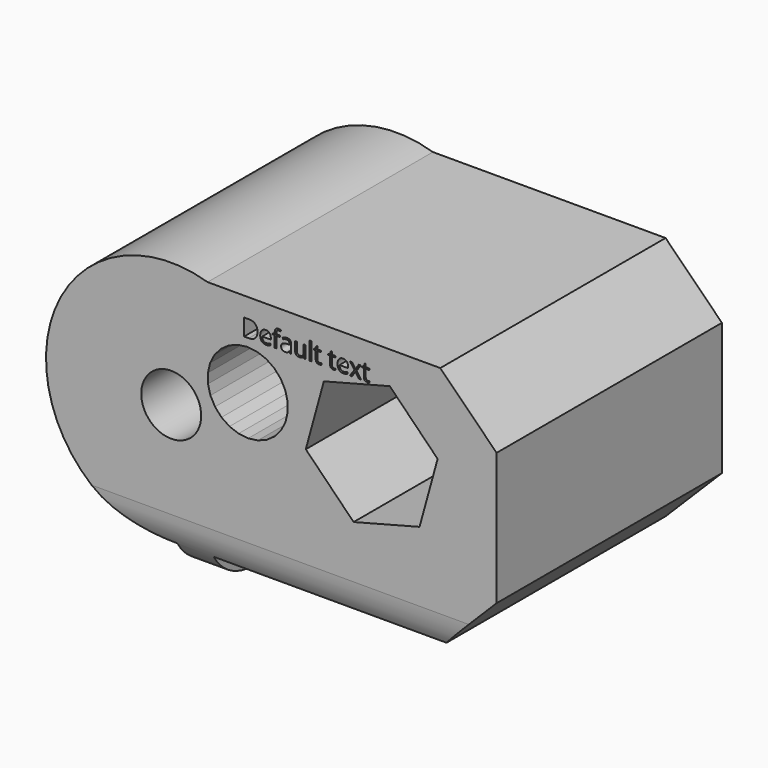
from build123d import *

# Parameters (mm, degrees)
F0_R     = 2.7024697733
F0_W     = 0.1718478913
F0_H     = 1.6102048079
F1_DEPTH = 25.4
F2_SIZE  = 5.08
F3_R     = 5.08


with BuildPart() as f1:
    # F0 (on Front) → F1 (new body)
    with BuildSketch(Plane.XZ):
        with BuildLine():
            Line((0, 2.5030102115), (0, 0))
            Line((0, 0), (3.2798051834, 0))
            Line((3.2798051834, 0), (3.2798051834, 2.5030102115))
            Line((3.2798051834, 2.5030102115), (29.3456315994, 2.5030102115))
            Line((29.3456315994, 2.5030102115), (29.3456315994, 24.5985444635))
            Line((29.3456315994, 24.5985444635), (3.2798051834, 24.5985444635))
            ThreePointArc((3.2798051834, 24.5985444635), (-11.168815469, 15.4520710292), (0, 2.5030102115))
        make_face()
        with Locations((0, 13.7942003278)):
            Circle(F0_R, mode=Mode.SUBTRACT)
        Polygon((9.9041786466, 14.9791304164), (9.3326310608, 14.3201610706), (8.6199899223, 13.8171204665), (7.8076713438, 13.4992434956), (6.9428843285, 13.385004012), (6.0758871541, 13.4810411992), (5.2570665453, 13.781773725), (4.5340093793, 14.2697241081), (3.9487371106, 14.9165344458), (3.5352636359, 15.6846144725), (3.3176185308, 16.5293261687), (3.3084505376, 17.4015779612), (3.5082924668, 18.2506777463), (3.9055302318, 19.0272789307), (4.4770778176, 19.6862482765), (5.1897189561, 20.1892888806), (6.0020375346, 20.5071658515), (6.8668245499, 20.6214053351), (7.7338217243, 20.5253681479), (8.5526423331, 20.2246356221), (9.2756994991, 19.736685239), (9.8609717678, 19.0898749012), (10.2744452425, 18.3217948746), (10.4920903476, 17.4770831783), (10.5012583408, 16.6048313858), (10.3014164116, 15.7557316008), align=None, mode=Mode.SUBTRACT)
        with BuildLine():
            add(Edge.make_bspline(
                [(8.7658543335, 21.3448248485), (8.6847315332, 21.327606948), (8.5698351589, 21.327606948)],
                knots=[0, 0, 0, 1, 1, 1], degree=2))
            add(Edge.make_bspline(
                [(8.5698351589, 21.327606948), (8.3185200347, 21.327606948), (8.1729956643, 21.480912485)],
                knots=[0, 0, 0, 1, 1, 1], degree=2))
            add(Edge.make_bspline(
                [(8.1729956643, 21.480912485), (8.0274712939, 21.6342180219), (8.0274712939, 21.9060621813)],
                knots=[0, 0, 0, 1, 1, 1], degree=2))
            add(Edge.make_bspline(
                [(8.0274712939, 21.9060621813), (8.0274712939, 22.1805552485), (8.16256559, 22.3419730654)],
                knots=[0, 0, 0, 1, 1, 1], degree=2))
            add(Edge.make_bspline(
                [(8.16256559, 22.3419730654), (8.297659886, 22.5033908824), (8.5254659538, 22.5033908824)],
                knots=[0, 0, 0, 1, 1, 1], degree=2))
            add(Edge.make_bspline(
                [(8.5254659538, 22.5033908824), (8.7383719155, 22.5033908824), (8.862539467, 22.3631643275)],
                knots=[0, 0, 0, 1, 1, 1], degree=2))
            add(Edge.make_bspline(
                [(8.862539467, 22.3631643275), (8.9867070185, 22.2229377727), (8.9867070185, 21.9931450241)],
                knots=[0, 0, 0, 1, 1, 1], degree=2))
            Line((8.9867070185, 21.9931450241), (8.9867070185, 21.8845398057))
            Line((8.9867070185, 21.8845398057), (8.2056103412, 21.8845398057))
            add(Edge.make_bspline(
                [(8.2056103412, 21.8845398057), (8.2109081567, 21.6848783829), (8.3065999497, 21.5814054233)],
                knots=[0, 0, 0, 1, 1, 1], degree=2))
            add(Edge.make_bspline(
                [(8.3065999497, 21.5814054233), (8.4022917427, 21.4779324637), (8.5761263148, 21.4779324637)],
                knots=[0, 0, 0, 1, 1, 1], degree=2))
            add(Edge.make_bspline(
                [(8.5761263148, 21.4779324637), (8.7592320641, 21.4779324637), (8.9380333383, 21.5544196754)],
                knots=[0, 0, 0, 1, 1, 1], degree=2))
            Line((8.9380333383, 21.5544196754), (8.9380333383, 21.4011141385))
            add(Edge.make_bspline(
                [(8.9380333383, 21.4011141385), (8.8469771338, 21.362042749), (8.7658543335, 21.3448248485)],
                knots=[0, 0, 0, 1, 1, 1], degree=2))
        make_face(mode=Mode.SUBTRACT)
        with BuildLine():
            add(Edge.make_bspline(
                [(7.5836136865, 22.6658020397), (7.7791361909, 22.4702795353), (7.7791361909, 22.1192992564)],
                knots=[0, 0, 0, 1, 1, 1], degree=2))
            add(Edge.make_bspline(
                [(7.7791361909, 22.1192992564), (7.7791361909, 21.7448099211), (7.57583252, 21.5466385089)],
                knots=[0, 0, 0, 1, 1, 1], degree=2))
            add(Edge.make_bspline(
                [(7.57583252, 21.5466385089), (7.372528849, 21.3484670967), (6.9907550173, 21.3484670967)],
                knots=[0, 0, 0, 1, 1, 1], degree=2))
            Line((6.9907550173, 21.3484670967), (6.5715653634, 21.3484670967))
            Line((6.5715653634, 21.3484670967), (6.5715653634, 22.8613245442))
            Line((6.5715653634, 22.8613245442), (7.0351242224, 22.8613245442))
            add(Edge.make_bspline(
                [(7.0351242224, 22.8613245442), (7.3880911821, 22.8613245442), (7.5836136865, 22.6658020397)],
                knots=[0, 0, 0, 1, 1, 1], degree=2))
        make_face(mode=Mode.SUBTRACT)
        Polygon((24.0267553463, 17.3061252721), (22.3968336872, 11.3822308036), (16.4516297587, 9.8318371323), (12.1363474891, 14.2053379295), (13.7662691482, 20.129232398), (19.7114730768, 21.6796260693), align=None, mode=Mode.SUBTRACT)
        with BuildLine():
            Line((10.8227312133, 21.3484670967), (10.6952525271, 21.3484670967))
            Line((10.6952525271, 21.3484670967), (10.6611478396, 21.5100504704))
            Line((10.6611478396, 21.5100504704), (10.6528700029, 21.5100504704))
            add(Edge.make_bspline(
                [(10.6528700029, 21.5100504704), (10.5681049544, 21.4034319328), (10.4838365761, 21.3655194404)],
                knots=[0, 0, 0, 1, 1, 1], degree=2))
            add(Edge.make_bspline(
                [(10.4838365761, 21.3655194404), (10.3995681978, 21.327606948), (10.273082852, 21.327606948)],
                knots=[0, 0, 0, 1, 1, 1], degree=2))
            add(Edge.make_bspline(
                [(10.273082852, 21.327606948), (10.1045460954, 21.327606948), (10.0088543024, 21.4146897908)],
                knots=[0, 0, 0, 1, 1, 1], degree=2))
            add(Edge.make_bspline(
                [(10.0088543024, 21.4146897908), (9.9131625094, 21.5017726336), (9.9131625094, 21.6620315534)],
                knots=[0, 0, 0, 1, 1, 1], degree=2))
            add(Edge.make_bspline(
                [(9.9131625094, 21.6620315534), (9.9131625094, 22.0053962225), (10.4624797572, 22.021951896)],
                knots=[0, 0, 0, 1, 1, 1], degree=2))
            Line((10.4624797572, 22.021951896), (10.6548566837, 22.028243052))
            Line((10.6548566837, 22.028243052), (10.6548566837, 22.0987702212))
            add(Edge.make_bspline(
                [(10.6548566837, 22.0987702212), (10.6548566837, 22.2322089499), (10.5975740533, 22.2957827363)],
                knots=[0, 0, 0, 1, 1, 1], degree=2))
            add(Edge.make_bspline(
                [(10.5975740533, 22.2957827363), (10.5402914228, 22.3593565226), (10.413806077, 22.3593565226)],
                knots=[0, 0, 0, 1, 1, 1], degree=2))
            add(Edge.make_bspline(
                [(10.413806077, 22.3593565226), (10.2720895116, 22.3593565226), (10.0932882374, 22.2726047933)],
                knots=[0, 0, 0, 1, 1, 1], degree=2))
            Line((10.0932882374, 22.2726047933), (10.0403100821, 22.4040568412))
            add(Edge.make_bspline(
                [(10.0403100821, 22.4040568412), (10.1240817902, 22.4494193867), (10.2239125016, 22.4752462374)],
                knots=[0, 0, 0, 1, 1, 1], degree=2))
            add(Edge.make_bspline(
                [(10.2239125016, 22.4752462374), (10.323743213, 22.5010730881), (10.4244017081, 22.5010730881)],
                knots=[0, 0, 0, 1, 1, 1], degree=2))
            add(Edge.make_bspline(
                [(10.4244017081, 22.5010730881), (10.6270431522, 22.5010730881), (10.7248871827, 22.4111757808)],
                knots=[0, 0, 0, 1, 1, 1], degree=2))
            add(Edge.make_bspline(
                [(10.7248871827, 22.4111757808), (10.8227312133, 22.3212784735), (10.8227312133, 22.1226103911)],
                knots=[0, 0, 0, 1, 1, 1], degree=2))
            Line((10.8227312133, 22.1226103911), (10.8227312133, 21.3484670967))
        make_face(mode=Mode.SUBTRACT)
        with BuildLine():
            Line((11.1641092016, 22.4825307337), (11.3379437737, 22.4825307337))
            Line((11.3379437737, 22.4825307337), (11.3379437737, 21.7467966019))
            add(Edge.make_bspline(
                [(11.3379437737, 21.7467966019), (11.3379437737, 21.6080600577), (11.4010208898, 21.5398506827)],
                knots=[0, 0, 0, 1, 1, 1], degree=2))
            add(Edge.make_bspline(
                [(11.4010208898, 21.5398506827), (11.464098006, 21.4716413078), (11.5985300751, 21.4716413078)],
                knots=[0, 0, 0, 1, 1, 1], degree=2))
            add(Edge.make_bspline(
                [(11.5985300751, 21.4716413078), (11.7766691223, 21.4716413078), (11.858785263, 21.5688231114)],
                knots=[0, 0, 0, 1, 1, 1], degree=2))
            add(Edge.make_bspline(
                [(11.858785263, 21.5688231114), (11.9409014038, 21.6660049151), (11.9409014038, 21.8865264865)],
                knots=[0, 0, 0, 1, 1, 1], degree=2))
            Line((11.9409014038, 21.8865264865), (11.9409014038, 22.4825307337))
            Line((11.9409014038, 22.4825307337), (12.112749295, 22.4825307337))
            Line((12.112749295, 22.4825307337), (12.112749295, 21.3484670967))
            Line((12.112749295, 21.3484670967), (11.9710327296, 21.3484670967))
            Line((11.9710327296, 21.3484670967), (11.9461992193, 21.5004481797))
            Line((11.9461992193, 21.5004481797), (11.9369280421, 21.5004481797))
            add(Edge.make_bspline(
                [(11.9369280421, 21.5004481797), (11.8842810003, 21.4166764716), (11.7905758881, 21.3721417098)],
                knots=[0, 0, 0, 1, 1, 1], degree=2))
            add(Edge.make_bspline(
                [(11.7905758881, 21.3721417098), (11.6968707759, 21.327606948), (11.576676586, 21.327606948)],
                knots=[0, 0, 0, 1, 1, 1], degree=2))
            add(Edge.make_bspline(
                [(11.576676586, 21.327606948), (11.3697306669, 21.327606948), (11.2669199342, 21.4259476488)],
                knots=[0, 0, 0, 1, 1, 1], degree=2))
            add(Edge.make_bspline(
                [(11.2669199342, 21.4259476488), (11.1641092016, 21.5242883496), (11.1641092016, 21.740505446)],
                knots=[0, 0, 0, 1, 1, 1], degree=2))
            Line((11.1641092016, 21.740505446), (11.1641092016, 22.4825307337))
        make_face(mode=Mode.SUBTRACT)
        with BuildLine():
            add(Edge.make_bspline(
                [(15.7347995507, 21.3448248485), (15.6536767503, 21.327606948), (15.538780376, 21.327606948)],
                knots=[0, 0, 0, 1, 1, 1], degree=2))
            add(Edge.make_bspline(
                [(15.538780376, 21.327606948), (15.2874652518, 21.327606948), (15.1419408814, 21.480912485)],
                knots=[0, 0, 0, 1, 1, 1], degree=2))
            add(Edge.make_bspline(
                [(15.1419408814, 21.480912485), (14.9964165111, 21.6342180219), (14.9964165111, 21.9060621813)],
                knots=[0, 0, 0, 1, 1, 1], degree=2))
            add(Edge.make_bspline(
                [(14.9964165111, 21.9060621813), (14.9964165111, 22.1805552485), (15.1315108071, 22.3419730654)],
                knots=[0, 0, 0, 1, 1, 1], degree=2))
            add(Edge.make_bspline(
                [(15.1315108071, 22.3419730654), (15.2666051031, 22.5033908824), (15.4944111709, 22.5033908824)],
                knots=[0, 0, 0, 1, 1, 1], degree=2))
            add(Edge.make_bspline(
                [(15.4944111709, 22.5033908824), (15.7073171326, 22.5033908824), (15.8314846841, 22.3631643275)],
                knots=[0, 0, 0, 1, 1, 1], degree=2))
            add(Edge.make_bspline(
                [(15.8314846841, 22.3631643275), (15.9556522356, 22.2229377727), (15.9556522356, 21.9931450241)],
                knots=[0, 0, 0, 1, 1, 1], degree=2))
            Line((15.9556522356, 21.9931450241), (15.9556522356, 21.8845398057))
            Line((15.9556522356, 21.8845398057), (15.1745555583, 21.8845398057))
            add(Edge.make_bspline(
                [(15.1745555583, 21.8845398057), (15.1798533738, 21.6848783829), (15.2755451668, 21.5814054233)],
                knots=[0, 0, 0, 1, 1, 1], degree=2))
            add(Edge.make_bspline(
                [(15.2755451668, 21.5814054233), (15.3712369599, 21.4779324637), (15.545071532, 21.4779324637)],
                knots=[0, 0, 0, 1, 1, 1], degree=2))
            add(Edge.make_bspline(
                [(15.545071532, 21.4779324637), (15.7281772812, 21.4779324637), (15.9069785554, 21.5544196754)],
                knots=[0, 0, 0, 1, 1, 1], degree=2))
            Line((15.9069785554, 21.5544196754), (15.9069785554, 21.4011141385))
            add(Edge.make_bspline(
                [(15.9069785554, 21.4011141385), (15.815922351, 21.362042749), (15.7347995507, 21.3448248485)],
                knots=[0, 0, 0, 1, 1, 1], degree=2))
        make_face(mode=Mode.SUBTRACT)
        Polygon((16.1069710917, 21.3484670967), (16.5218562704, 21.9289090108), (16.1275001269, 22.4825307337), (16.323188188, 22.4825307337), (16.622183652, 22.0481098602), (16.9201857756, 22.4825307337), (17.113887156, 22.4825307337), (16.7195310124, 21.9289090108), (17.1344161912, 21.3484670967), (16.9400525839, 21.3484670967), (16.622183652, 21.808052594), (16.301334699, 21.3484670967), align=None, mode=Mode.SUBTRACT)
        with BuildLine():
            Line((9.7909816387, 22.4825307337), (9.7909816387, 22.349092005))
            Line((9.7909816387, 22.349092005), (9.5022506923, 22.349092005))
            Line((9.5022506923, 22.349092005), (9.5022506923, 21.3484670967))
            Line((9.5022506923, 21.3484670967), (9.330402801, 21.3484670967))
            Line((9.330402801, 21.3484670967), (9.330402801, 22.349092005))
            Line((9.330402801, 22.349092005), (9.127761357, 22.349092005))
            Line((9.127761357, 22.349092005), (9.127761357, 22.4265725572))
            Line((9.127761357, 22.4265725572), (9.330402801, 22.4888218897))
            Line((9.330402801, 22.4888218897), (9.330402801, 22.5517334491))
            add(Edge.make_bspline(
                [(9.330402801, 22.5517334491), (9.330402801, 22.9699297625), (9.6956209592, 22.9699297625)],
                knots=[0, 0, 0, 1, 1, 1], degree=2))
            add(Edge.make_bspline(
                [(9.6956209592, 22.9699297625), (9.7856838232, 22.9699297625), (9.9068713535, 22.9338383942)],
                knots=[0, 0, 0, 1, 1, 1], degree=2))
            Line((9.9068713535, 22.9338383942), (9.8621710349, 22.7960951904))
            add(Edge.make_bspline(
                [(9.8621710349, 22.7960951904), (9.7628369937, 22.8282131971), (9.6926409379, 22.8282131971)],
                knots=[0, 0, 0, 1, 1, 1], degree=2))
            add(Edge.make_bspline(
                [(9.6926409379, 22.8282131971), (9.5952935776, 22.8282131971), (9.5487721349, 22.7634805136)],
                knots=[0, 0, 0, 1, 1, 1], degree=2))
            add(Edge.make_bspline(
                [(9.5487721349, 22.7634805136), (9.5022506923, 22.6987478301), (9.5022506923, 22.5560379242)],
                knots=[0, 0, 0, 1, 1, 1], degree=2))
            Line((9.5022506923, 22.5560379242), (9.5022506923, 22.4825307337))
            Line((9.5022506923, 22.4825307337), (9.7909816387, 22.4825307337))
        make_face(mode=Mode.SUBTRACT)
        with Locations((12.5628980584, 22.1535695006)):
            Rectangle(F0_W, F0_H, mode=Mode.SUBTRACT)
        with BuildLine():
            add(Edge.make_bspline(
                [(13.2458195917, 21.5244539063), (13.2944932718, 21.469654627), (13.3792583203, 21.469654627)],
                knots=[0, 0, 0, 1, 1, 1], degree=2))
            add(Edge.make_bspline(
                [(13.3792583203, 21.469654627), (13.4249519793, 21.469654627), (13.4673345035, 21.4762768964)],
                knots=[0, 0, 0, 1, 1, 1], degree=2))
            add(Edge.make_bspline(
                [(13.4673345035, 21.4762768964), (13.5097170278, 21.4828991658), (13.5345505381, 21.4901836621)],
                knots=[0, 0, 0, 1, 1, 1], degree=2))
            Line((13.5345505381, 21.4901836621), (13.5345505381, 21.3587316143))
            add(Edge.make_bspline(
                [(13.5345505381, 21.3587316143), (13.5067370065, 21.3454870755), (13.4524343973, 21.3365470117)],
                knots=[0, 0, 0, 1, 1, 1], degree=2))
            add(Edge.make_bspline(
                [(13.4524343973, 21.3365470117), (13.3981317882, 21.327606948), (13.35442481, 21.327606948)],
                knots=[0, 0, 0, 1, 1, 1], degree=2))
            add(Edge.make_bspline(
                [(13.35442481, 21.327606948), (13.0256291337, 21.327606948), (13.0256291337, 21.6742827518)],
                knots=[0, 0, 0, 1, 1, 1], degree=2))
            Line((13.0256291337, 21.6742827518), (13.0256291337, 22.349092005))
            Line((13.0256291337, 22.349092005), (12.8630524196, 22.349092005))
            Line((12.8630524196, 22.349092005), (12.8630524196, 22.4318703727))
            Line((12.8630524196, 22.4318703727), (13.0256291337, 22.5033908824))
            Line((13.0256291337, 22.5033908824), (13.0978118703, 22.7454348294))
            Line((13.0978118703, 22.7454348294), (13.1971459115, 22.7454348294))
            Line((13.1971459115, 22.7454348294), (13.1971459115, 22.4825307337))
            Line((13.1971459115, 22.4825307337), (13.5262727013, 22.4825307337))
            Line((13.5262727013, 22.4825307337), (13.5262727013, 22.349092005))
            Line((13.5262727013, 22.349092005), (13.1971459115, 22.349092005))
            Line((13.1971459115, 22.349092005), (13.1971459115, 21.6815672482))
            add(Edge.make_bspline(
                [(13.1971459115, 21.6815672482), (13.1971459115, 21.5792531857), (13.2458195917, 21.5244539063)],
                knots=[0, 0, 0, 1, 1, 1], degree=2))
        make_face(mode=Mode.SUBTRACT)
        with BuildLine():
            add(Edge.make_bspline(
                [(14.5444466236, 21.5244539063), (14.5931203038, 21.469654627), (14.6778853523, 21.469654627)],
                knots=[0, 0, 0, 1, 1, 1], degree=2))
            add(Edge.make_bspline(
                [(14.6778853523, 21.469654627), (14.7235790112, 21.469654627), (14.7659615355, 21.4762768964)],
                knots=[0, 0, 0, 1, 1, 1], degree=2))
            add(Edge.make_bspline(
                [(14.7659615355, 21.4762768964), (14.8083440597, 21.4828991658), (14.83317757, 21.4901836621)],
                knots=[0, 0, 0, 1, 1, 1], degree=2))
            Line((14.83317757, 21.4901836621), (14.83317757, 21.3587316143))
            add(Edge.make_bspline(
                [(14.83317757, 21.3587316143), (14.8053640385, 21.3454870755), (14.7510614293, 21.3365470117)],
                knots=[0, 0, 0, 1, 1, 1], degree=2))
            add(Edge.make_bspline(
                [(14.7510614293, 21.3365470117), (14.6967588201, 21.327606948), (14.653051842, 21.327606948)],
                knots=[0, 0, 0, 1, 1, 1], degree=2))
            add(Edge.make_bspline(
                [(14.653051842, 21.327606948), (14.3242561656, 21.327606948), (14.3242561656, 21.6742827518)],
                knots=[0, 0, 0, 1, 1, 1], degree=2))
            Line((14.3242561656, 21.6742827518), (14.3242561656, 22.349092005))
            Line((14.3242561656, 22.349092005), (14.1616794515, 22.349092005))
            Line((14.1616794515, 22.349092005), (14.1616794515, 22.4318703727))
            Line((14.1616794515, 22.4318703727), (14.3242561656, 22.5033908824))
            Line((14.3242561656, 22.5033908824), (14.3964389022, 22.7454348294))
            Line((14.3964389022, 22.7454348294), (14.4957729434, 22.7454348294))
            Line((14.4957729434, 22.7454348294), (14.4957729434, 22.4825307337))
            Line((14.4957729434, 22.4825307337), (14.8248997333, 22.4825307337))
            Line((14.8248997333, 22.4825307337), (14.8248997333, 22.349092005))
            Line((14.8248997333, 22.349092005), (14.4957729434, 22.349092005))
            Line((14.4957729434, 22.349092005), (14.4957729434, 21.6815672482))
            add(Edge.make_bspline(
                [(14.4957729434, 21.6815672482), (14.4957729434, 21.5792531857), (14.5444466236, 21.5244539063)],
                knots=[0, 0, 0, 1, 1, 1], degree=2))
        make_face(mode=Mode.SUBTRACT)
        with BuildLine():
            add(Edge.make_bspline(
                [(17.5916838942, 21.5244539063), (17.6403575743, 21.469654627), (17.7251226228, 21.469654627)],
                knots=[0, 0, 0, 1, 1, 1], degree=2))
            add(Edge.make_bspline(
                [(17.7251226228, 21.469654627), (17.7708162818, 21.469654627), (17.813198806, 21.4762768964)],
                knots=[0, 0, 0, 1, 1, 1], degree=2))
            add(Edge.make_bspline(
                [(17.813198806, 21.4762768964), (17.8555813303, 21.4828991658), (17.8804148406, 21.4901836621)],
                knots=[0, 0, 0, 1, 1, 1], degree=2))
            Line((17.8804148406, 21.4901836621), (17.8804148406, 21.3587316143))
            add(Edge.make_bspline(
                [(17.8804148406, 21.3587316143), (17.852601309, 21.3454870755), (17.7982986998, 21.3365470117)],
                knots=[0, 0, 0, 1, 1, 1], degree=2))
            add(Edge.make_bspline(
                [(17.7982986998, 21.3365470117), (17.7439960907, 21.327606948), (17.7002891125, 21.327606948)],
                knots=[0, 0, 0, 1, 1, 1], degree=2))
            add(Edge.make_bspline(
                [(17.7002891125, 21.327606948), (17.3714934362, 21.327606948), (17.3714934362, 21.6742827518)],
                knots=[0, 0, 0, 1, 1, 1], degree=2))
            Line((17.3714934362, 21.6742827518), (17.3714934362, 22.349092005))
            Line((17.3714934362, 22.349092005), (17.2089167221, 22.349092005))
            Line((17.2089167221, 22.349092005), (17.2089167221, 22.4318703727))
            Line((17.2089167221, 22.4318703727), (17.3714934362, 22.5033908824))
            Line((17.3714934362, 22.5033908824), (17.4436761728, 22.7454348294))
            Line((17.4436761728, 22.7454348294), (17.543010214, 22.7454348294))
            Line((17.543010214, 22.7454348294), (17.543010214, 22.4825307337))
            Line((17.543010214, 22.4825307337), (17.8721370038, 22.4825307337))
            Line((17.8721370038, 22.4825307337), (17.8721370038, 22.349092005))
            Line((17.8721370038, 22.349092005), (17.543010214, 22.349092005))
            Line((17.543010214, 22.349092005), (17.543010214, 21.6815672482))
            add(Edge.make_bspline(
                [(17.543010214, 21.6815672482), (17.543010214, 21.5792531857), (17.5916838942, 21.5244539063)],
                knots=[0, 0, 0, 1, 1, 1], degree=2))
        make_face(mode=Mode.SUBTRACT)
    extrude(amount=F1_DEPTH)

    # F2
    f2_edges = [f1.edges().sort_by_distance(p)[0] for p in [
        (29.345632, -12.7, 24.598544),
        (29.345632, -12.7, 2.50301),
    ]]
    chamfer(f2_edges, length=F2_SIZE)

    # F3
    f3_edges = [f1.edges().sort_by_distance(p)[0] for p in [
        (1.639903, -25.4, 0),
    ]]
    fillet(f3_edges, radius=F3_R)


solid = f1.part
